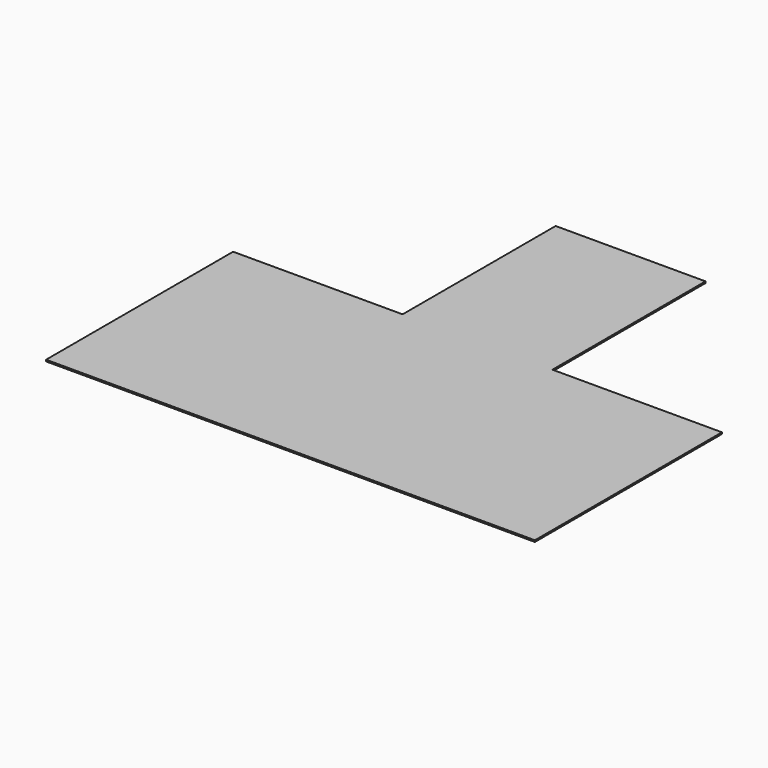
from build123d import *

# Parameters (mm, degrees)
F1_DEPTH = 1.4111111111
F2_DEPTH = 101.2317
F3_DEPTH = 66.675
F4_DEPTH = 66.675
F5_DEPTH = 47.498


# Not quite as in the source:
# - a length typed as a fraction of an inch, garbled in the dataset ("3 / 203.2 mm" for 3/8 in), is restored


with BuildPart() as f1:
    # F0 (on Top) → F1 (new body)
    with BuildSketch(Plane.XY):
        Polygon((-156.2699383586, 189.0532364881), (-290.5952983586, 189.0532364881), (-290.5952983586, -36.1571907997), (-375.8326183586, -36.1571907997), (-375.8326183586, -144.4919435119), (-71.0326183586, -144.4919435119), (-71.0326183586, -36.1571907997), (-156.2699383586, -36.1571907997), align=None)
    extrude(amount=F1_DEPTH)

    # F2 (add): faces of the model
    f2_faces = [f1.faces().sort_by_distance(p)[0] for p in [
        (-333.2139583586, -36.1571907997, 0.7055555556),
        (-113.6512783586, -36.1571907997, 0.7055555556),
    ]]
    extrude(f2_faces, amount=F2_DEPTH)

    # F3 (add): a face of the model
    f3_faces = [f1.faces().sort_by_distance(p)[0] for p in [
        (-71.0326183586, -39.7087171558, 0.7055555556),
    ]]
    extrude(f3_faces, amount=F3_DEPTH)

    # F4 (add): a face of the model
    f4_faces = [f1.faces().sort_by_distance(p)[0] for p in [
        (-375.8326183586, -39.7087171558, 0.7055555556),
    ]]
    extrude(f4_faces, amount=F4_DEPTH)

    # F5 (add): a face of the model
    f5_faces = [f1.faces().sort_by_distance(p)[0] for p in [
        (-223.4326183586, 189.0532364881, 0.7055555556),
    ]]
    extrude(f5_faces, amount=F5_DEPTH)


solid = f1.part
